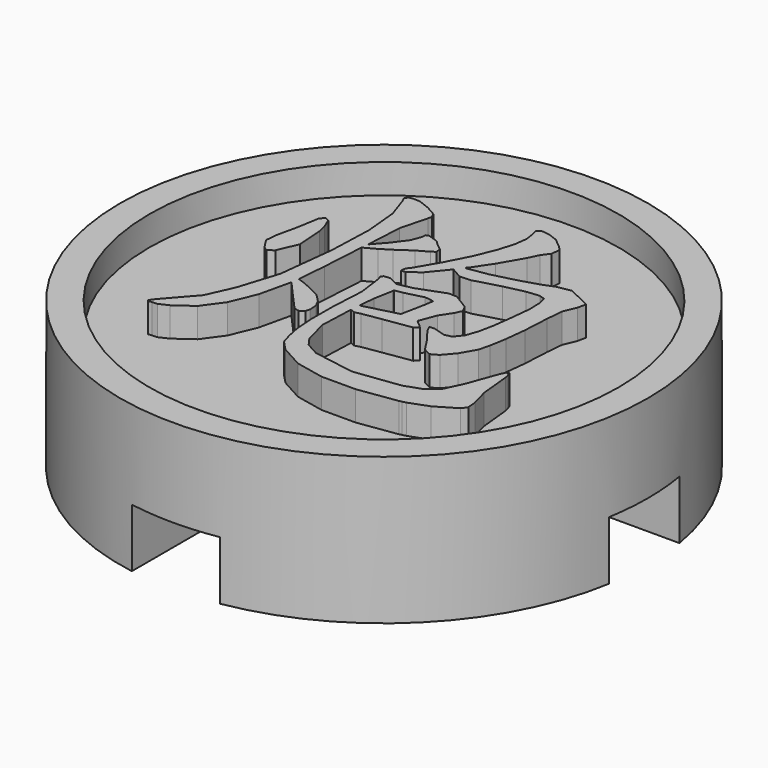
from build123d import *

# Parameters (mm, degrees)
F0_R     = 9
F1_DEPTH = 4
F3_W     = 3
F3_H     = 3
F4_DEPTH = 2
F2_R     = 9
F2_R_2   = 8
F5_DEPTH = 1
F7_DEPTH = 1


# Not quite as in the source:
# - a feature names something its author has since deleted; it is built from what else it names


with BuildPart() as f1:
    # F0 (on Top) → F1 (new body)
    with BuildSketch(Plane.XY):
        with Locations((-31.3306450844, 19.7580661625)):
            Circle(F0_R)
    extrude(amount=F1_DEPTH)

    # F3 (on face) → F4 (cut)
    with BuildSketch(Plane(origin=(0, 0, 0), x_dir=(1, 0, 0), z_dir=(0, 0, -1))):
        with BuildLine():
            ThreePointArc((-32.8306450844, -28.6321858371), (-32.0832814269, -28.7265408676), (-31.3306450844, -28.7580661625))
            ThreePointArc((-31.3306450844, -28.7580661625), (-30.5780087419, -28.7265408676), (-29.8306450844, -28.6321858371))
            Line((-29.8306450844, -28.6321858371), (-29.8306450844, -21.2580661625))
            Line((-29.8306450844, -21.2580661625), (-32.8306450844, -21.2580661625))
            Line((-32.8306450844, -21.2580661625), (-32.8306450844, -28.6321858371))
        make_face()
        with BuildLine():
            ThreePointArc((-40.204764759, -18.2580661625), (-40.2991197895, -19.0054298199), (-40.3306450844, -19.7580661625))
            ThreePointArc((-40.3306450844, -19.7580661625), (-40.2991197895, -20.510702505), (-40.204764759, -21.2580661625))
            Line((-40.204764759, -21.2580661625), (-32.8306450844, -21.2580661625))
            Line((-32.8306450844, -21.2580661625), (-32.8306450844, -18.2580661625))
            Line((-32.8306450844, -18.2580661625), (-40.204764759, -18.2580661625))
        make_face()
        with Locations((-31.3306450844, -19.7580661625)):
            Rectangle(F3_W, F3_H)
        with BuildLine():
            Line((-29.8306450844, -18.2580661625), (-29.8306450844, -21.2580661625))
            Line((-29.8306450844, -21.2580661625), (-22.4565254097, -21.2580661625))
            ThreePointArc((-22.4565254097, -21.2580661625), (-22.3621703793, -20.510702505), (-22.3306450844, -19.7580661625))
            ThreePointArc((-22.3306450844, -19.7580661625), (-22.3621703793, -19.0054298199), (-22.4565254097, -18.2580661625))
            Line((-22.4565254097, -18.2580661625), (-29.8306450844, -18.2580661625))
        make_face()
        with BuildLine():
            Line((-32.8306450844, -10.8839464878), (-32.8306450844, -18.2580661625))
            Line((-32.8306450844, -18.2580661625), (-29.8306450844, -18.2580661625))
            Line((-29.8306450844, -18.2580661625), (-29.8306450844, -10.8839464878))
            ThreePointArc((-29.8306450844, -10.8839464878), (-30.5780087419, -10.7895914574), (-31.3306450844, -10.7580661625))
            ThreePointArc((-31.3306450844, -10.7580661625), (-32.0832814269, -10.7895914574), (-32.8306450844, -10.8839464878))
        make_face()
    extrude(amount=-F4_DEPTH, mode=Mode.SUBTRACT)

    # F2 (on face) → F5 (join)
    with BuildSketch(Plane.XY.offset(4)):
        with Locations((-31.3306450844, 19.7580661625)):
            Circle(F2_R)
        with Locations((-31.3306450844, 19.7580661625)):
            Circle(F2_R_2, mode=Mode.SUBTRACT)
    extrude(amount=F5_DEPTH)

    # F6 (on face) → F7 (join)
    with BuildSketch(Plane.XY.offset(4)):
        Polygon((-31.535583115, 21.6900881108), (-31.0133508406, 22.3245785838), (-30.6411076918, 22.1117900598), (-30.2594389346, 22.1298548595), (-29.3760303382, 22.3756387116), (-28.7084875503, 22.5264256518), (-28.2687208016, 22.5735536939), (-28.0700649916, 22.5068222098), (-28.0111406922, 22.224053957), (-27.9978057928, 21.8000155513), (-28.0763335341, 21.0563384655), (-28.1579955466, 20.4430356662), (-28.2601158024, 19.9459345484), (-28.3998473131, 19.5477795245), (-28.614231466, 19.280785204), (-28.8490738622, 19.2210972822), (-29.2637094542, 19.3436073971), (-29.4498281793, 19.3389059902), (-29.3610998098, 19.1488437821), (-28.9865259029, 18.6509790419), (-28.72655235, 18.2473361939), (-28.4603672414, 18.1099069479), (-28.2177176605, 18.2473361939), (-27.8964833515, 18.6258478852), (-27.6083013574, 19.1237126254), (-27.5124496442, 19.503814247), (-27.4174527322, 20.0590190549), (-27.3381841631, 20.779895742), (-27.291056121, 21.6555541404), (-27.2376595363, 22.2389844855), (-27.0585501815, 22.6638207057), (-26.9988850544, 22.952857501), (-27.2776642347, 23.0949824552), (-27.7779509118, 23.3329591226), (-28.2647887159, 23.2449715808), (-28.65115888, 23.0965780842), (-29.3108374964, 22.8931353872), (-30.1047768955, 22.6929409349), (-30.8186043216, 22.5790244219), (-30.8217385929, 22.5986848506), (-30.7683477069, 22.654417892), (-30.3482242909, 23.2818989947), (-29.895065656, 24.0617056799), (-29.7286073596, 24.409552801), (-29.5432864491, 24.6585279112), (-29.5055612207, 24.963179076), (-29.6673466035, 25.1280987301), (-29.9579220411, 25.365277583), (-30.2759650921, 25.4877990952), (-30.5390159294, 25.5223330656), (-30.685095764, 25.4139442674), (-30.636406285, 25.2176819008), (-30.5908510771, 24.9192422918), (-30.6434840393, 24.4998767996), (-30.8076058789, 23.9439140679), (-31.0981642204, 23.2355687671), (-31.4868879373, 22.4816910531), (-31.9243068319, 21.7277563524), (-32.0295271668, 21.5887656695), (-32.0593597304, 21.5079014715), (-32.0601461475, 21.4019061167), (-31.9148755248, 21.4105111159), align=None)
        Polygon((-31.1845504345, 20.8144866991), (-31.6824208734, 20.7162985291), (-31.9871290249, 20.876488283), (-32.216432309, 20.863951198), (-32.2808216377, 20.7822891854), (-32.2289978874, 20.6315022453), (-32.1190476522, 19.7928054529), (-32.1818755439, 18.6352734936), (-32.1857962323, 17.7306088395), (-32.1379045677, 17.0630888463), (-32.0467998507, 16.6170478565), (-31.9368724102, 16.251882462), (-31.6227500476, 15.922846667), (-30.8633560163, 15.5050654064), (-29.8958634705, 15.3016728577), (-28.7360121505, 15.302458705), (-27.4009835614, 15.4956454966), (-27.3295221771, 15.5152717333), (-27.1936657654, 15.5459021113), (-26.5512541342, 15.785417421), (-25.8680969769, 16.1898466861), (-25.7408455644, 16.3665398027), (-25.7707066213, 16.6767357783), (-25.934828461, 17.2861178893), (-26.0376895445, 18.3195668994), (-26.0754147729, 18.4703481408), (-26.1224858283, 18.5865840145), (-26.2018113841, 18.548106561), (-26.2701384971, 18.4169515562), (-26.6596429325, 17.3505129166), (-26.951813999, 16.7364123027), (-27.3193215489, 16.4427139913), (-27.9004154373, 16.2369633309), (-29.4545580795, 16.0367118919), (-30.8657095691, 16.2746600659), (-31.3094141022, 16.5188881798), (-31.5253710895, 16.8212256825), (-31.7405359609, 17.6457954597), (-31.6949807531, 18.8064559915), (-31.5395038034, 18.7436337985), (-31.3400330829, 18.7938961119), (-30.7102269207, 18.8944093413), (-29.76314133, 19.0389163416), (-29.6280827329, 19.1582750892), (-29.7184067314, 19.2454420217), (-29.9076597277, 19.4032953189), (-29.6846135887, 19.9914897563), (-29.4333020218, 20.3644908288), (-29.3194424956, 20.6087303401), (-29.4333020218, 20.8262259696), (-29.9579220411, 21.1560652778), (-30.2508339354, 21.162390807), (-30.6835286284, 20.9990097952), align=None)
        Polygon((-31.6203793988, 19.6985607659), (-31.5002399328, 20.3267997925), (-31.5002399328, 20.3896219855), (-31.226167858, 20.4383114646), (-30.5987095499, 20.5969511789), (-30.4314249457, 20.5859527361), (-30.2940298918, 20.5466888655), (-30.3411579339, 20.2380600256), (-30.5013476878, 19.4409920539), (-31.6698552951, 19.1363009984), align=None, mode=Mode.SUBTRACT)
        Polygon((-35.5272485026, 22.5193592948), (-35.6497586175, 22.3717066259), (-35.7777594057, 21.6248952689), (-35.9293225054, 20.9362103968), (-35.969373363, 20.5333425687), (-35.7471330167, 20.1823098882), (-35.5994963041, 20.0810102416), (-35.4078840564, 20.2200066232), (-35.1141800462, 20.9032150687), (-35.1754351037, 21.8125526362), (-35.2578949307, 22.1369212165), (-35.3827528997, 22.447100096), align=None)
        Polygon((-34.1694651043, 17.9701241492), (-33.9221084179, 19.0514819199), (-33.7273448029, 18.8315871482), (-33.0080124567, 18.0274414222), (-32.9145541869, 17.9284896297), (-32.7535837146, 17.8829572166), (-32.5965111359, 17.9897446872), (-32.554112994, 18.1326845519), (-32.5713799792, 18.4043859779), (-32.6876044556, 18.639194182), (-32.9483245349, 18.9038406484), (-33.5985604469, 19.2210972822), (-33.8844116828, 19.3184762404), (-33.8035132927, 20.3103135257), (-33.7147792245, 21.7780186658), (-33.3205676837, 21.9932006333), (-32.9860212699, 22.2021140583), (-32.5006993134, 22.5350876378), (-32.1316132305, 22.7392141758), (-32.0051824273, 22.83347026), (-32.021668694, 23.0031198144), (-32.1975753935, 23.1405148683), (-32.3892047373, 23.3203650509), (-32.7410181362, 23.4397522918), (-32.8321057572, 23.3988927922), (-32.82581442, 23.2952338942), (-32.9640243845, 22.9269285298), (-33.3127035122, 22.4596941677), (-33.6896480678, 22.032464504), (-33.6221187692, 23.2897631662), (-33.3849570123, 24.196764277), (-33.35825872, 24.3294864175), (-33.4352193257, 24.4888783568), (-33.7705464579, 24.6765927109), (-34.1545459732, 24.8281204788), (-34.4058404441, 24.838321107), (-34.5440561072, 24.8155833938), (-34.609231853, 24.6977917818), (-34.553476017, 24.5988057973), (-34.2927616363, 23.8323909984), (-34.1851649539, 22.6960752061), (-34.2385786346, 21.174927892), (-34.4561027575, 19.2556540473), (-34.8848767621, 17.8986570662), (-35.2853796402, 17.0065579905), (-36.1492064496, 16.0202199265), (-36.2591487066, 15.8600244739), (-36.2371603692, 15.823114156), (-36.111511994, 15.8380332871), (-35.9293225054, 15.8474588956), (-35.6152018524, 15.9950944684), (-35.0168067867, 16.4238627744), (-34.5346304988, 17.088220003), align=None)
    extrude(amount=F7_DEPTH)


solid = f1.part
